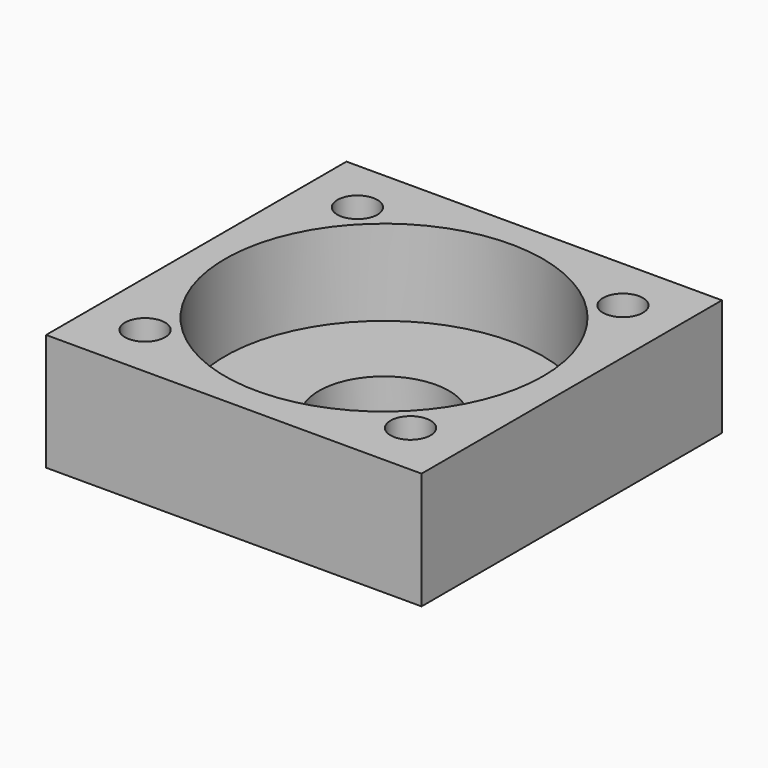
from build123d import *

# Parameters (mm, degrees)
F0_W     = 38.1
F0_H     = 38.1
F0_R     = 2.032
F0_R_2   = 16.129
F1_DEPTH = 8.6868
F2_W     = 38.1
F2_H     = 38.1
F2_R     = 6.604
F3_DEPTH = 3.175
F4_DEPTH = 3.175


# Not quite as in the source:
# - a feature of the source that left no trace in its solid (it failed there, or was rolled back) is left out


with BuildPart() as f1:
    # F0 (on Top) → F1 (new body)
    with BuildSketch(Plane.XY):
        Rectangle(F0_W, F0_H)
        with Locations((-13.4688665365, -13.4719016558)):
            Circle(F0_R, mode=Mode.SUBTRACT)
        with Locations((13.4729134635, -13.4719016558)):
            Circle(F0_R, mode=Mode.SUBTRACT)
        with Locations((-13.47089, 13.4698783442)):
            Circle(F0_R, mode=Mode.SUBTRACT)
        Circle(F0_R_2, mode=Mode.SUBTRACT)
        with Locations((13.47089, 13.4698783442)):
            Circle(F0_R, mode=Mode.SUBTRACT)
    extrude(amount=F1_DEPTH)

    # F2 (on Top) → F3 (join)
    with BuildSketch(Plane.XY):
        Rectangle(F2_W, F2_H)
        Circle(F2_R, mode=Mode.SUBTRACT)
    extrude(amount=-F3_DEPTH)

    # F4 (cut, through all): faces of the model
    f4_faces = [f1.faces().sort_by_distance(p)[0] for p in [
        (-13.47089, 13.4698783442, 0),
        (-13.4688665365, -13.4719016558, 0),
        (13.4729134635, -13.4719016558, 0),
        (13.47089, 13.4698783442, 0),
    ]]
    extrude(f4_faces, amount=-F4_DEPTH, mode=Mode.SUBTRACT)


solid = f1.part
